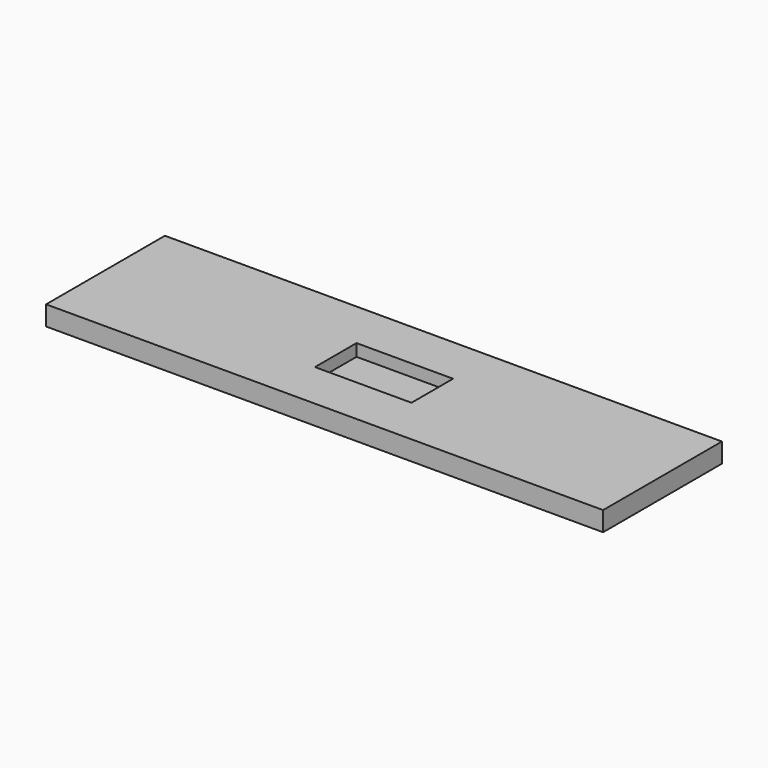
from build123d import *

# Parameters (mm, degrees)
F1_DEPTH = 6.6802
F2_DEPTH = 2.54
F3_DEPTH = 6.6802


with BuildPart() as f1:
    # F0 (on Top) → F1 (new body)
    with BuildSketch(Plane.XY):
        Polygon((-95.25, -25.4), (95.25, -25.4), (95.25, 0), (95.25, 25.4), (-95.25, 25.4), align=None)
        Polygon((22.225, 22.225), (22.225, 0), (22.225, -22.225), (-22.225, -22.225), (-22.225, 22.225), align=None, mode=Mode.SUBTRACT)
    extrude(amount=F1_DEPTH)


with BuildPart() as f2:
    # F0 (on Top) → F2 (new body)
    with BuildSketch(Plane.XY):
        Polygon((16.51, -8.89), (16.51, 0), (16.51, 8.89), (-16.51, 8.89), (-16.51, -8.89), align=None)
    extrude(amount=F2_DEPTH)

    # F0 (on Top) → F3 (join)
    with BuildSketch(Plane.XY):
        Polygon((-95.25, -25.4), (95.25, -25.4), (95.25, 0), (95.25, 25.4), (-95.25, 25.4), align=None)
        Polygon((22.225, 22.225), (22.225, 0), (22.225, -22.225), (-22.225, -22.225), (-22.225, 22.225), align=None, mode=Mode.SUBTRACT)
        Polygon((22.225, -22.225), (22.225, 0), (22.225, 22.225), (-22.225, 22.225), (-22.225, -22.225), align=None)
        Polygon((16.51, 8.89), (16.51, 0), (16.51, -8.89), (-16.51, -8.89), (-16.51, 8.89), align=None, mode=Mode.SUBTRACT)
    extrude(amount=F3_DEPTH)


solid = Compound([f1.part, f2.part])
